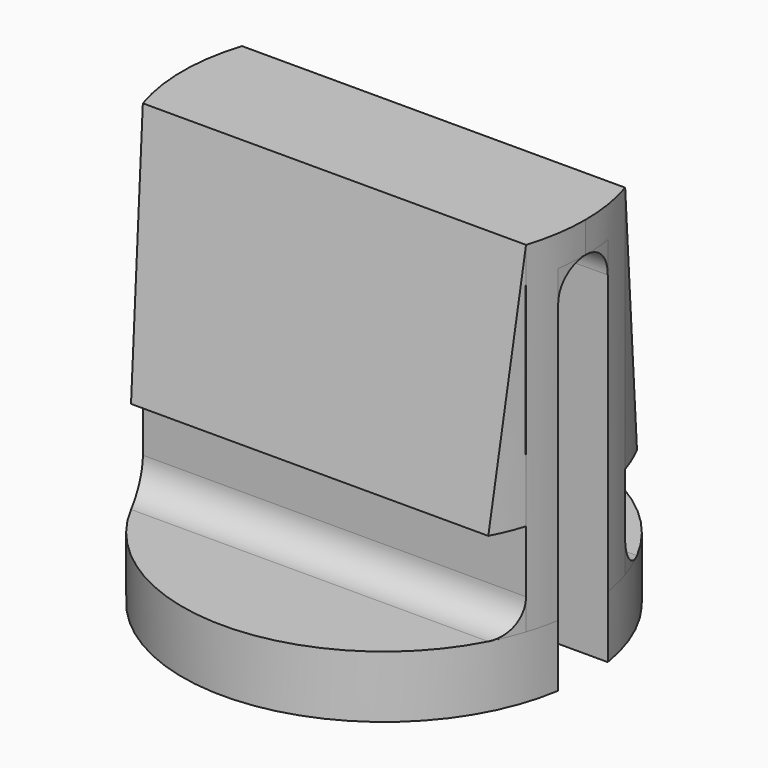
from build123d import *
from build123d import SkipClean  # not in build123d's __all__

# Parameters (mm, degrees)
F0_R          = 6.5
F1_DEPTH      = 1
F3_DEPTH      = 11
F7_R          = 1.375
F8_DEPTH      = 12
F9_W          = 46.4800073215
F9_H          = 2
F10_DEPTH     = 12
F11_T4_DEPTH  = 10.4788869849
F11_S5_R      = 1.375
F11_T6_DEPTH  = 7
F11_S7_R      = 6.5
F11_T8_DEPTH  = 7
F11_T12_DEPTH = 10.4788869849
F11_S13_R     = 6.5
F11_T14_DEPTH = 7
F11_S15_R     = 1.375
F11_T16_DEPTH = 7
F11_T20_DEPTH = 10.4788869849
F11_S21_R     = 1.375
F11_T22_DEPTH = 7
F11_S23_R     = 6.5
F11_T24_DEPTH = 7
F11_T28_DEPTH = 10.4788869849
F11_S29_R     = 1.375
F11_T30_DEPTH = 7
F11_S31_R     = 6.5
F11_T32_DEPTH = 7
F11_T36_DEPTH = 17.3693168769
F11_S37_R     = 6.5
F11_T38_DEPTH = 10
F11_T42_DEPTH = 17.3693168769
F11_S43_R     = 6.5
F11_T44_DEPTH = 10


# Not quite as in the source:
# - a fillet or chamfer that OpenCascade refuses, or shapes differently, is made with other operations: its cross-section is extruded or revolved along the edge and cut away or added
# - after a boolean that leaves OpenCascade's solid faulty, fix() repairs it


with BuildPart() as f1:
    # F0 (on Top) → F1 (new body, symmetric)
    with BuildSketch(Plane.XY):
        Circle(F0_R)
    extrude(amount=F1_DEPTH, both=True)

    # F2 (on face) → F3 (join)
    with BuildSketch(Plane.XY.offset(1)):
        with BuildLine():
            ThreePointArc((6.5, 0), (6.4206806434, 1.0123537302), (6.1846584384, 2))
            Line((6.1846584384, 2), (-6.1846584384, 2))
            ThreePointArc((-6.1846584384, 2), (-6.5, 0), (-6.1846584384, -2))
            Line((-6.1846584384, -2), (6.1846584384, -2))
            ThreePointArc((6.1846584384, -2), (6.4206806434, -1.0123537302), (6.5, 0))
        make_face()
    with SkipClean():  # cleaning this boolean's faces spoils the solid; the shape is the same uncleaned
        extrude(amount=F3_DEPTH)

    # F5 (on offset) → F6 section 0
    with BuildSketch(Plane.XY.offset(4)):
        with BuildLine():
            ThreePointArc((5.7662812973, -3), (6.5, 0), (5.7662812973, 3))
            Line((5.7662812973, 3), (-5.7662812973, 3))
            ThreePointArc((-5.7662812973, 3), (-6.5, 0), (-5.7662812973, -3))
            Line((-5.7662812973, -3), (5.7662812973, -3))
        make_face()
    # F3_face (on face) → F6 section 1
    with BuildSketch(Plane.XY.offset(12)):
        with BuildLine():
            ThreePointArc((6.1846584384, -2), (6.5, 0), (6.1846584384, 2))
            Line((6.1846584384, 2), (-6.1846584384, 2))
            ThreePointArc((-6.1846584384, 2), (-6.5, 0), (-6.1846584384, -2))
            Line((-6.1846584384, -2), (6.1846584384, -2))
        make_face()
    loft()

    add(f1.part.fix(), mode=Mode.REPLACE)

    # F7 (on face) → F8 (cut)
    with BuildSketch(Plane(origin=(0, 0, -1), x_dir=(1, 0, 0), z_dir=(0, 0, -1))):
        Circle(F7_R)
    extrude(amount=-F8_DEPTH, mode=Mode.SUBTRACT)

    # F9 (on face) → F10 (cut)
    with BuildSketch(Plane(origin=(0, 0, -1), x_dir=(1, 0, 0), z_dir=(0, 0, -1))):
        Rectangle(F9_W, F9_H)
    extrude(amount=-F10_DEPTH, mode=Mode.SUBTRACT)

    # F11: fillet of radius 1 on 8 edges, made by hand


with BuildPart() as f11_tool2:
    # F11_s3 → F11_t4 (new body)
    with BuildSketch(Plane.YZ.offset(-8.9226162893)):
        with BuildLine():
            ThreePointArc((0, 11), (0.7071067812, 10.7071067812), (1, 10))
            Line((1, 10), (1, 11))
            Line((1, 11), (0, 11))
        make_face()
    extrude(amount=F11_T4_DEPTH)

    # F11_s5 → F11_t6 (cut, symmetric)
    with BuildSketch(Plane.XY.offset(10.5)):
        Circle(F11_S5_R)
    extrude(amount=F11_T6_DEPTH, both=True, mode=Mode.SUBTRACT)

    # F11_s7 → F11_t8 (intersect, symmetric)
    with BuildSketch(Plane.XY.offset(10.5)):
        Circle(F11_S7_R)
    extrude(amount=F11_T8_DEPTH, both=True, mode=Mode.INTERSECT)


with BuildPart() as f1_1:
    add(f1.part, clean=False)

    # F11_t1: union F11_tool2
    add(f11_tool2.part)


with BuildPart() as f11_tool10:
    # F11_s11 → F11_t12 (new body)
    with BuildSketch(Plane.YZ.offset(-1.5562706956)):
        with BuildLine():
            ThreePointArc((1, 10), (0.7071067812, 10.7071067812), (0, 11))
            Line((0, 11), (1, 11))
            Line((1, 11), (1, 10))
        make_face()
    extrude(amount=F11_T12_DEPTH)

    # F11_s13 → F11_t14 (intersect, symmetric)
    with BuildSketch(Plane.XY.offset(10.5)):
        Circle(F11_S13_R)
    extrude(amount=F11_T14_DEPTH, both=True, mode=Mode.INTERSECT)

    # F11_s15 → F11_t16 (cut, symmetric)
    with BuildSketch(Plane.XY.offset(10.5)):
        Circle(F11_S15_R)
    extrude(amount=F11_T16_DEPTH, both=True, mode=Mode.SUBTRACT)


with BuildPart() as f1_2:
    add(f1_1.part, clean=False)

    # F11_t9: union F11_tool10
    add(f11_tool10.part)


with BuildPart() as f11_tool18:
    # F11_s19 → F11_t20 (new body)
    with BuildSketch(Plane.YZ.offset(8.9226162893)):
        with BuildLine():
            ThreePointArc((-1, 10), (-0.7071067812, 10.7071067812), (0, 11))
            Line((0, 11), (-1, 11))
            Line((-1, 11), (-1, 10))
        make_face()
    extrude(amount=-F11_T20_DEPTH)

    # F11_s21 → F11_t22 (cut, symmetric)
    with BuildSketch(Plane.XY.offset(10.5)):
        Circle(F11_S21_R)
    extrude(amount=F11_T22_DEPTH, both=True, mode=Mode.SUBTRACT)

    # F11_s23 → F11_t24 (intersect, symmetric)
    with BuildSketch(Plane.XY.offset(10.5)):
        Circle(F11_S23_R)
    extrude(amount=F11_T24_DEPTH, both=True, mode=Mode.INTERSECT)


with BuildPart() as f1_3:
    add(f1_2.part, clean=False)

    # F11_t17: union F11_tool18
    add(f11_tool18.part)


with BuildPart() as f11_tool26:
    # F11_s27 → F11_t28 (new body)
    with BuildSketch(Plane.YZ.offset(1.5562706956)):
        with BuildLine():
            ThreePointArc((0, 11), (-0.7071067812, 10.7071067812), (-1, 10))
            Line((-1, 10), (-1, 11))
            Line((-1, 11), (0, 11))
        make_face()
    extrude(amount=-F11_T28_DEPTH)

    # F11_s29 → F11_t30 (cut, symmetric)
    with BuildSketch(Plane.XY.offset(10.5)):
        Circle(F11_S29_R)
    extrude(amount=F11_T30_DEPTH, both=True, mode=Mode.SUBTRACT)

    # F11_s31 → F11_t32 (intersect, symmetric)
    with BuildSketch(Plane.XY.offset(10.5)):
        Circle(F11_S31_R)
    extrude(amount=F11_T32_DEPTH, both=True, mode=Mode.INTERSECT)


with BuildPart() as f1_4:
    add(f1_3.part, clean=False)

    # F11_t25: union F11_tool26
    add(f11_tool26.part)


with BuildPart() as f11_tool34:
    # F11_s35 → F11_t36 (new body)
    with BuildSketch(Plane.YZ.offset(8.6846584384)):
        with BuildLine():
            ThreePointArc((3, 1), (2.2928932188, 1.2928932188), (2, 2))
            Line((2, 2), (2, 1))
            Line((2, 1), (3, 1))
        make_face()
    extrude(amount=-F11_T36_DEPTH)

    # F11_s37 → F11_t38 (intersect, symmetric)
    with BuildSketch(Plane.XY.offset(1.5)):
        Circle(F11_S37_R)
    extrude(amount=F11_T38_DEPTH, both=True, mode=Mode.INTERSECT)


with BuildPart() as f1_5:
    add(f1_4.part, clean=False)

    # F11_t33: union F11_tool34
    add(f11_tool34.part)


with BuildPart() as f11_tool40:
    # F11_s41 → F11_t42 (new body)
    with BuildSketch(Plane.YZ.offset(-8.6846584384)):
        with BuildLine():
            ThreePointArc((-2, 2), (-2.2928932188, 1.2928932188), (-3, 1))
            Line((-3, 1), (-2, 1))
            Line((-2, 1), (-2, 2))
        make_face()
    extrude(amount=F11_T42_DEPTH)

    # F11_s43 → F11_t44 (intersect, symmetric)
    with BuildSketch(Plane.XY.offset(1.5)):
        Circle(F11_S43_R)
    extrude(amount=F11_T44_DEPTH, both=True, mode=Mode.INTERSECT)


with BuildPart() as f1_6:
    add(f1_5.part, clean=False)

    # F11_t39: union F11_tool40
    add(f11_tool40.part)


solid = f1_6.part
